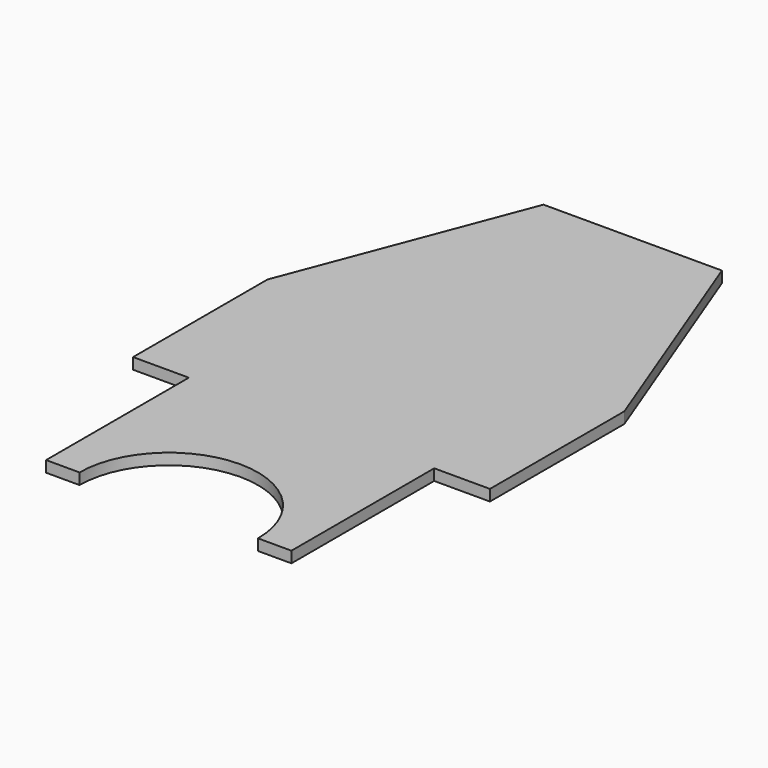
from build123d import *

# Parameters (mm, degrees)
F1_DEPTH = 3.175


# Not quite as in the source:
# - a length typed as a fraction of an inch, garbled in the dataset ("3 / 203.2 mm" for 3/8 in), is restored


with BuildPart() as f1:
    # F0 (on Top) → F1 (new body)
    with BuildSketch(Plane.XY):
        with BuildLine():
            Line((50.8, 0), (25.4, 66.475))
            Line((25.4, 66.475), (-25.4, 66.475))
            Line((-25.4, 66.475), (-50.8, 0))
            Line((-50.8, 0), (-50.8, -47.825))
            Line((-50.8, -47.825), (-34.925, -47.825))
            Line((-34.925, -47.825), (-34.925, -98.625))
            Line((-34.925, -98.625), (-25.4, -98.625))
            ThreePointArc((-25.4, -98.625), (0, -73.225), (25.4, -98.625))
            Line((25.4, -98.625), (34.925, -98.625))
            Line((34.925, -98.625), (34.925, -47.825))
            Line((34.925, -47.825), (50.8, -47.825))
            Line((50.8, -47.825), (50.8, 0))
        make_face()
    extrude(amount=-F1_DEPTH)


solid = f1.part
